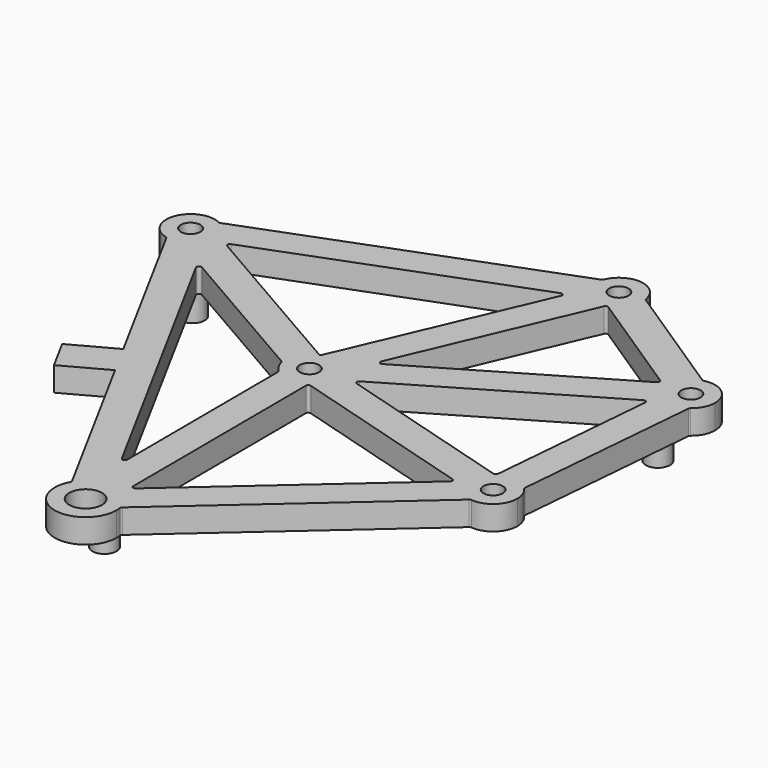
from build123d import *

# Parameters (mm, degrees)
F1_R        = 0.8
F1_R_2      = 1.35
F2_DEPTH    = 2
F3_R        = 1
F4_DEPTH    = 5
F5_T1_DEPTH = 2


# Not quite as in the source:
# - a fillet or chamfer that OpenCascade refuses, or shapes differently, is made with other operations: its cross-section is extruded or revolved along the edge and cut away or added


with BuildPart() as f2:
    # F1 (on Top) → F2 (new body)
    with BuildSketch(Plane.XY):
        with BuildLine():
            ThreePointArc((5.1588517672, 41.7551647468), (5.8189357702, 41.1743283067), (6.1661273036, 40.3665288884))
            Line((6.1661273036, 40.3665288884), (7.2214972283, 39.7576616241))
            Line((7.2214972283, 39.7576616241), (28.9007343827, 47.9973716865))
            Line((28.9007343827, 47.9973716865), (29.5069198348, 49.4140747655))
            ThreePointArc((29.5069198348, 49.4140747655), (29.3032782438, 50.1855350347), (29.4174253255, 50.9752129996))
            Line((29.4174253255, 50.9752129996), (5.1588517672, 41.7551647468))
        make_face()
        with BuildLine():
            Line((43.2422348913, 44.0206504324), (33.2838919458, 50.5533234047))
            ThreePointArc((33.2838919458, 50.5533234047), (33.2959689241, 50.4269175094), (33.3, 50.3))
            ThreePointArc((33.3, 50.3), (32.9116112847, 49.1156398068), (31.8972909329, 48.3912717476))
            Line((31.8972909329, 48.3912717476), (31.8846447163, 48.361716545))
            Line((31.8846447163, 48.361716545), (41.3390492003, 42.1596272035))
            Line((41.3390492003, 42.1596272035), (41.8307045309, 42.4491065103))
            ThreePointArc((41.8307045309, 42.4491065103), (42.3120664109, 43.4364331761), (43.2422348913, 44.0206504324))
        make_face()
        with BuildLine():
            Line((43.6267783824, 25.1015361028), (44.9634471469, 40.4732268946))
            ThreePointArc((44.9634471469, 40.4732268946), (44.0887539119, 40.1209544779), (43.1498718292, 40.2086160195))
            Line((43.1498718292, 40.2086160195), (42.2864184602, 39.7002275873))
            Line((42.2864184602, 39.7002275873), (41.0423751405, 25.3937294107))
            Line((41.0423751405, 25.3937294107), (41.1068738191, 25.3748358584))
            ThreePointArc((41.1068738191, 25.3748358584), (42.4156481787, 25.6883399767), (43.6267783824, 25.1015361028))
        make_face()
        with BuildLine():
            Line((23.7876337156, 9.1717796898), (23.790532231, 8.4993241145))
            ThreePointArc((23.790532231, 8.4993241145), (24.5837459945, 7.769864834), (25.0048179717, 6.7778984503))
            Line((25.0048179717, 6.7778984503), (41.9214502868, 21.7194924748))
            ThreePointArc((41.9214502868, 21.7194924748), (40.9992832251, 22.1005378321), (40.3759708626, 22.8796843864))
            Line((40.3759708626, 22.8796843864), (39.5736067493, 23.1147203388))
            Line((39.5736067493, 23.1147203388), (23.7876337156, 9.1717796898))
        make_face()
        with BuildLine():
            ThreePointArc((6.0825746745, 39.3247870004), (6.1704249985, 39.6573262113), (6.2, 40))
            ThreePointArc((6.2, 40), (6.1915138221, 40.184045365), (6.1661273036, 40.3665288884))
            ThreePointArc((6.1661273036, 40.3665288884), (5.8189357702, 41.1743283067), (5.1588517672, 41.7551647468))
            ThreePointArc((5.1588517672, 41.7551647468), (2.3247456616, 40.6952849534), (3.782863546, 38.0439843613))
            ThreePointArc((3.782863546, 38.0439843613), (4.3297316575, 38.004212011), (4.8668489245, 38.1144463646))
            ThreePointArc((4.8668489245, 38.1144463646), (5.5958497172, 38.5676580133), (6.0677200026, 39.2847224372))
            ThreePointArc((6.0677200026, 39.2847224372), (6.0752543384, 39.3047150466), (6.0825746745, 39.3247870004))
        make_face()
        with Locations((4.2, 40)):
            Circle(F1_R, mode=Mode.SUBTRACT)
        with BuildLine():
            ThreePointArc((33.2838919458, 50.5533234047), (31.5169424001, 52.2881991839), (29.4174253255, 50.9752129996))
            ThreePointArc((29.4174253255, 50.9752129996), (29.3032782438, 50.1855350347), (29.5069198348, 49.4140747655))
            ThreePointArc((29.5069198348, 49.4140747655), (29.8570250617, 48.9151450158), (30.3411482328, 48.5448352532))
            ThreePointArc((30.3411482328, 48.5448352532), (31.0830575999, 48.3118008161), (31.8577651087, 48.3793495676))
            ThreePointArc((31.8577651087, 48.3793495676), (31.8775587843, 48.3852086666), (31.8972909329, 48.3912717476))
            ThreePointArc((31.8972909329, 48.3912717476), (32.9116112847, 49.1156398068), (33.3, 50.3))
            ThreePointArc((33.3, 50.3), (33.2959689241, 50.4269175094), (33.2838919458, 50.5533234047))
        make_face()
        with Locations((31.3, 50.3)):
            Circle(F1_R, mode=Mode.SUBTRACT)
        with BuildLine():
            ThreePointArc((45.8, 42.1), (45.0009308437, 43.699301444), (43.2422348913, 44.0206504324))
            ThreePointArc((43.2422348913, 44.0206504324), (42.3120664109, 43.4364331761), (41.8307045309, 42.4491065103))
            ThreePointArc((41.8307045309, 42.4491065103), (41.8005868024, 42.1484444539), (41.8161080542, 41.8466765953))
            ThreePointArc((41.8161080542, 41.8466765953), (42.0006206287, 41.2269399345), (42.3732216176, 40.6984638972))
            ThreePointArc((42.3732216176, 40.6984638972), (42.7330543859, 40.4083655665), (43.1498718292, 40.2086160195))
            ThreePointArc((43.1498718292, 40.2086160195), (44.0887539119, 40.1209544779), (44.9634471469, 40.4732268946))
            ThreePointArc((44.9634471469, 40.4732268946), (45.578608205, 41.1853673671), (45.8, 42.1))
        make_face()
        with Locations((43.8, 42.1)):
            Circle(F1_R, mode=Mode.SUBTRACT)
        with BuildLine():
            ThreePointArc((44.2, 23.7), (44.0511559584, 24.4571140057), (43.6267783824, 25.1015361028))
            ThreePointArc((43.6267783824, 25.1015361028), (42.4156481787, 25.6883399767), (41.1068738191, 25.3748358584))
            ThreePointArc((41.1068738191, 25.3748358584), (41.071457443, 25.351178881), (41.0365528531, 25.3267731054))
            ThreePointArc((41.0365528531, 25.3267731054), (40.4141774879, 24.6004654104), (40.2002527524, 23.6682046258))
            ThreePointArc((40.2002527524, 23.6682046258), (40.2478838399, 23.2649798885), (40.3759708626, 22.8796843864))
            ThreePointArc((40.3759708626, 22.8796843864), (40.9992832251, 22.1005378321), (41.9214502868, 21.7194924748))
            ThreePointArc((41.9214502868, 21.7194924748), (43.512040505, 22.1905134273), (44.2, 23.7))
        make_face()
        with Locations((42.2, 23.7)):
            Circle(F1_R, mode=Mode.SUBTRACT)
        with BuildLine():
            ThreePointArc((22.5955597255, 8.8482088491), (21.8669162755, 8.7701629496), (21.1905563835, 8.4881173221))
            ThreePointArc((21.1905563835, 8.4881173221), (20.6960652476, 8.1023094654), (20.3107032689, 7.6074707733))
            ThreePointArc((20.3107032689, 7.6074707733), (21.8218431835, 3.8418292711), (25.05, 6.3))
            ThreePointArc((25.05, 6.3), (25.0386793641, 6.5400147623), (25.0048179717, 6.7778984503))
            ThreePointArc((25.0048179717, 6.7778984503), (24.5837459945, 7.769864834), (23.790532231, 8.4993241145))
            ThreePointArc((23.790532231, 8.4993241145), (23.5432842899, 8.6268128181), (23.2836204373, 8.7266106013))
            ThreePointArc((23.2836204373, 8.7266106013), (22.9437746873, 8.8110882157), (22.5955597255, 8.8482088491))
        make_face()
        with Locations((22.5, 6.3)):
            Circle(F1_R_2, mode=Mode.SUBTRACT)
        with BuildLine():
            Line((7.2214972283, 39.7576616241), (6.0825746745, 39.3247870004))
            ThreePointArc((6.0825746745, 39.3247870004), (6.0752543384, 39.3047150466), (6.0677200026, 39.2847224372))
            Line((6.0677200026, 39.2847224372), (7.5409732288, 36.5716823429))
            Line((7.5409732288, 36.5716823429), (20.4338726964, 29.1334711116))
            ThreePointArc((20.4338726964, 29.1334711116), (20.6676288279, 30.499444907), (21.7331510755, 31.3855536354))
            Line((21.7331510755, 31.3855536354), (7.2214972283, 39.7576616241))
        make_face()
        with BuildLine():
            ThreePointArc((6.1661273036, 40.3665288884), (6.1915138221, 40.184045365), (6.2, 40))
            ThreePointArc((6.2, 40), (6.1704249985, 39.6573262113), (6.0825746745, 39.3247870004))
            Line((6.0825746745, 39.3247870004), (7.2214972283, 39.7576616241))
            Line((7.2214972283, 39.7576616241), (6.1661273036, 40.3665288884))
        make_face()
        with BuildLine():
            Line((7.5409732288, 36.5716823429), (6.0677200026, 39.2847224372))
            ThreePointArc((6.0677200026, 39.2847224372), (5.5958497172, 38.5676580133), (4.8668489245, 38.1144463646))
            Line((4.8668489245, 38.1144463646), (7.5409732288, 36.5716823429))
        make_face()
        with BuildLine():
            ThreePointArc((4.8668489245, 38.1144463646), (4.3297316575, 38.004212011), (3.782863546, 38.0439843613))
            Line((3.782863546, 38.0439843613), (11.3309729791, 24.1439139846))
            Line((11.3309729791, 24.1439139846), (12.7625938358, 21.5075411501))
            Line((12.7625938358, 21.5075411501), (20.3107032689, 7.6074707733))
            ThreePointArc((20.3107032689, 7.6074707733), (20.6960652476, 8.1023094654), (21.1905563835, 8.4881173221))
            Line((21.1905563835, 8.4881173221), (21.1777502182, 11.4591476685))
            Line((21.1777502182, 11.4591476685), (7.5409732288, 36.5716823429))
            Line((7.5409732288, 36.5716823429), (4.8668489245, 38.1144463646))
        make_face()
        with BuildLine():
            Line((22.5955597255, 8.8482088491), (21.1777502182, 11.4591476685))
            Line((21.1777502182, 11.4591476685), (21.1905563835, 8.4881173221))
            ThreePointArc((21.1905563835, 8.4881173221), (21.8669162755, 8.7701629496), (22.5955597255, 8.8482088491))
        make_face()
        with BuildLine():
            Line((23.7876337156, 9.1717796898), (23.2836204373, 8.7266106013))
            ThreePointArc((23.2836204373, 8.7266106013), (23.5432842899, 8.6268128181), (23.790532231, 8.4993241145))
            Line((23.790532231, 8.4993241145), (23.7876337156, 9.1717796898))
        make_face()
        with BuildLine():
            Line((21.1065631723, 27.9745423071), (21.1777502182, 11.4591476685))
            Line((21.1777502182, 11.4591476685), (22.5955597255, 8.8482088491))
            ThreePointArc((22.5955597255, 8.8482088491), (22.9437746873, 8.8110882157), (23.2836204373, 8.7266106013))
            Line((23.2836204373, 8.7266106013), (23.7876337156, 9.1717796898))
            Line((23.7876337156, 9.1717796898), (23.7075018728, 27.7623672218))
            Line((23.7075018728, 27.7623672218), (23.4931261809, 27.8251641416))
            ThreePointArc((23.4931261809, 27.8251641416), (22.2750618238, 27.5039062016), (21.1065631723, 27.9745423071))
        make_face()
        with BuildLine():
            Line((40.2002527524, 23.6682046258), (39.5736067493, 23.1147203388))
            Line((39.5736067493, 23.1147203388), (40.3759708626, 22.8796843864))
            ThreePointArc((40.3759708626, 22.8796843864), (40.2478838399, 23.2649798885), (40.2002527524, 23.6682046258))
        make_face()
        with BuildLine():
            ThreePointArc((41.0365528531, 25.3267731054), (41.071457443, 25.351178881), (41.1068738191, 25.3748358584))
            Line((41.1068738191, 25.3748358584), (41.0423751405, 25.3937294107))
            Line((41.0423751405, 25.3937294107), (41.0365528531, 25.3267731054))
        make_face()
        with BuildLine():
            Line((29.5069198348, 49.4140747655), (28.9007343827, 47.9973716865))
            Line((28.9007343827, 47.9973716865), (30.3411482328, 48.5448352532))
            ThreePointArc((30.3411482328, 48.5448352532), (29.8570250617, 48.9151450158), (29.5069198348, 49.4140747655))
        make_face()
        with BuildLine():
            ThreePointArc((31.8972909329, 48.3912717476), (31.8775587843, 48.3852086666), (31.8577651087, 48.3793495676))
            Line((31.8577651087, 48.3793495676), (31.8846447163, 48.361716545))
            Line((31.8846447163, 48.361716545), (31.8972909329, 48.3912717476))
        make_face()
        with BuildLine():
            ThreePointArc((23.7065390199, 27.9857490995), (23.602516175, 27.9018902263), (23.4931261809, 27.8251641416))
            Line((23.4931261809, 27.8251641416), (23.7075018728, 27.7623672218))
            Line((23.7075018728, 27.7623672218), (23.7065390199, 27.9857490995))
        make_face()
        with BuildLine():
            Line((30.3411482328, 48.5448352532), (28.9007343827, 47.9973716865))
            Line((28.9007343827, 47.9973716865), (21.8027090671, 31.4087282524))
            ThreePointArc((21.8027090671, 31.4087282524), (22.4278055637, 31.4998067033), (23.0501281708, 31.3913839805))
            Line((23.0501281708, 31.3913839805), (25.1531087237, 32.6295874836))
            Line((25.1531087237, 32.6295874836), (31.8846447163, 48.361716545))
            Line((31.8846447163, 48.361716545), (31.8577651087, 48.3793495676))
            ThreePointArc((31.8577651087, 48.3793495676), (31.0830575999, 48.3118008161), (30.3411482328, 48.5448352532))
        make_face()
        with BuildLine():
            Line((25.1531087237, 32.6295874836), (23.0501281708, 31.3913839805))
            ThreePointArc((23.0501281708, 31.3913839805), (23.7210047561, 31.0016479062), (24.1930801652, 30.3859252345))
            Line((24.1930801652, 30.3859252345), (25.1531087237, 32.6295874836))
        make_face()
        with BuildLine():
            ThreePointArc((21.8027090671, 31.4087282524), (21.7678238691, 31.397459707), (21.7331510755, 31.3855536354))
            ThreePointArc((21.7331510755, 31.3855536354), (20.6676288279, 30.499444907), (20.4338726964, 29.1334711116))
            ThreePointArc((20.4338726964, 29.1334711116), (20.6702692189, 28.4959923182), (21.1065631723, 27.9745423071))
            ThreePointArc((21.1065631723, 27.9745423071), (22.2750618238, 27.5039062016), (23.4931261809, 27.8251641416))
            ThreePointArc((23.4931261809, 27.8251641416), (23.602516175, 27.9018902263), (23.7065390199, 27.9857490995))
            ThreePointArc((23.7065390199, 27.9857490995), (24.138437017, 28.5111437224), (24.3692954691, 29.1508934897))
            ThreePointArc((24.3692954691, 29.1508934897), (24.3923090797, 29.3247729161), (24.4, 29.5))
            ThreePointArc((24.4, 29.5), (24.3555124999, 29.9194888111), (24.2240291374, 30.3203156136))
            ThreePointArc((24.2240291374, 30.3203156136), (24.208852145, 30.353260756), (24.1930801652, 30.3859252345))
            ThreePointArc((24.1930801652, 30.3859252345), (23.7210047561, 31.0016479062), (23.0501281708, 31.3913839805))
            ThreePointArc((23.0501281708, 31.3913839805), (22.4278055637, 31.4998067033), (21.8027090671, 31.4087282524))
        make_face()
        with Locations((22.4, 29.5)):
            Circle(F1_R, mode=Mode.SUBTRACT)
        with BuildLine():
            ThreePointArc((24.3692954691, 29.1508934897), (24.138437017, 28.5111437224), (23.7065390199, 27.9857490995))
            Line((23.7065390199, 27.9857490995), (23.7075018728, 27.7623672218))
            Line((23.7075018728, 27.7623672218), (39.5736067493, 23.1147203388))
            Line((39.5736067493, 23.1147203388), (40.2002527524, 23.6682046258))
            ThreePointArc((40.2002527524, 23.6682046258), (40.4141774879, 24.6004654104), (41.0365528531, 25.3267731054))
            Line((41.0365528531, 25.3267731054), (41.0423751405, 25.3937294107))
            Line((41.0423751405, 25.3937294107), (25.6473390591, 29.9033864446))
            Line((25.6473390591, 29.9033864446), (24.3692954691, 29.1508934897))
        make_face()
        with BuildLine():
            Line((25.6473390591, 29.9033864446), (24.2240291374, 30.3203156136))
            ThreePointArc((24.2240291374, 30.3203156136), (24.3555124999, 29.9194888111), (24.4, 29.5))
            ThreePointArc((24.4, 29.5), (24.3923090797, 29.3247729161), (24.3692954691, 29.1508934897))
            Line((24.3692954691, 29.1508934897), (25.6473390591, 29.9033864446))
        make_face()
        with BuildLine():
            Line((25.1531087237, 32.6295874836), (24.1930801652, 30.3859252345))
            ThreePointArc((24.1930801652, 30.3859252345), (24.208852145, 30.353260756), (24.2240291374, 30.3203156136))
            Line((24.2240291374, 30.3203156136), (25.6473390591, 29.9033864446))
            Line((25.6473390591, 29.9033864446), (42.2864184602, 39.7002275873))
            Line((42.2864184602, 39.7002275873), (42.3732216176, 40.6984638972))
            ThreePointArc((42.3732216176, 40.6984638972), (42.0006206287, 41.2269399345), (41.8161080542, 41.8466765953))
            Line((41.8161080542, 41.8466765953), (41.3390492003, 42.1596272035))
            Line((41.3390492003, 42.1596272035), (25.1531087237, 32.6295874836))
        make_face()
        with BuildLine():
            ThreePointArc((41.8161080542, 41.8466765953), (41.8005868024, 42.1484444539), (41.8307045309, 42.4491065103))
            Line((41.8307045309, 42.4491065103), (41.3390492003, 42.1596272035))
            Line((41.3390492003, 42.1596272035), (41.8161080542, 41.8466765953))
        make_face()
        with BuildLine():
            Line((42.2864184602, 39.7002275873), (43.1498718292, 40.2086160195))
            ThreePointArc((43.1498718292, 40.2086160195), (42.7330543859, 40.4083655665), (42.3732216176, 40.6984638972))
            Line((42.3732216176, 40.6984638972), (42.2864184602, 39.7002275873))
        make_face()
        Polygon((12.7625938358, 21.5075411501), (11.3309729791, 24.1439139846), (7.8158091997, 22.2350861756), (9.2474300564, 19.5987133411), align=None)
    extrude(amount=-F2_DEPTH)

    # F3 (on face) → F4 (join)
    with BuildSketch(Plane.XY):
        with Locations((21.6236830238, 9.3353357393)):
            Circle(F3_R)
        with Locations((5.9410208844, 38.0202536185)):
            Circle(F3_R)
        with Locations((41.960581314, 40.9868787588)):
            Circle(F3_R)
    extrude(amount=-F4_DEPTH)

    # F5: fillet of radius 0.2 on 26 edges, made by hand

    # F5_s2 → F5_t1 (join)
    with BuildSketch(Plane.XY.offset(-2)):
        with BuildLine():
            ThreePointArc((7.6152873474, 39.9073309314), (7.4869831486, 39.736368397), (7.586398465, 39.5471416799))
            Line((7.586398465, 39.5471416799), (7.2214972283, 39.7576616241))
            Line((7.2214972283, 39.7576616241), (7.6152873474, 39.9073309314))
        make_face()
        with BuildLine():
            ThreePointArc((8.1549136009, 36.2174859744), (7.9153841385, 36.1874830559), (7.8792109212, 35.9488074668))
            Line((7.8792109212, 35.9488074668), (7.5409732288, 36.5716823429))
            Line((7.5409732288, 36.5716823429), (8.1549136009, 36.2174859744))
        make_face()
        with BuildLine():
            ThreePointArc((20.7985689859, 12.157421304), (21.0239808003, 12.0591244239), (21.174325317, 12.2537247554))
            Line((21.174325317, 12.2537247554), (21.1777502182, 11.4591476685))
            Line((21.1777502182, 11.4591476685), (20.7985689859, 12.157421304))
        make_face()
        with BuildLine():
            ThreePointArc((23.7857330682, 9.6127298888), (23.9039049915, 9.4310968268), (24.1181310207, 9.463691015))
            Line((24.1181310207, 9.463691015), (23.7876337156, 9.1717796898))
            Line((23.7876337156, 9.1717796898), (23.7857330682, 9.6127298888))
        make_face()
        with BuildLine():
            ThreePointArc((20.2576640938, 7.7051440082), (20.2819058756, 7.6098108546), (20.2577672936, 7.5144515183))
            ThreePointArc((20.2577672936, 7.5144515183), (20.2837472088, 7.5612389011), (20.3107032689, 7.6074707733))
            Line((20.3107032689, 7.6074707733), (20.2576640938, 7.7051440082))
        make_face()
        with BuildLine():
            ThreePointArc((25.0881216817, 6.8514763464), (25.0326730948, 6.7702265564), (25.0226653835, 6.6723699273))
            ThreePointArc((25.0226653835, 6.6723699273), (25.0142953862, 6.7252278342), (25.0048179717, 6.7778984503))
            Line((25.0048179717, 6.7778984503), (25.0881216817, 6.8514763464))
        make_face()
        with BuildLine():
            ThreePointArc((21.0426824665, 28.0310925443), (21.090007357, 27.9647639806), (21.1069488553, 27.8850638597))
            Line((21.1069488553, 27.8850638597), (21.1065631723, 27.9745423071))
            ThreePointArc((21.1065631723, 27.9745423071), (21.0743212482, 28.0024767625), (21.0426824665, 28.0310925443))
        make_face()
        with BuildLine():
            ThreePointArc((20.356367035, 29.1781859163), (20.4171704433, 29.1239450721), (20.4512932221, 29.0499534537))
            ThreePointArc((20.4512932221, 29.0499534537), (20.442137576, 29.0916193824), (20.4338726964, 29.1334711116))
            Line((20.4338726964, 29.1334711116), (20.356367035, 29.1781859163))
        make_face()
        with BuildLine():
            ThreePointArc((3.6998231735, 38.0635539919), (3.77290973, 38.0275334575), (3.8255636798, 37.9653507815))
            Line((3.8255636798, 37.9653507815), (3.782863546, 38.0439843613))
            ThreePointArc((3.782863546, 38.0439843613), (3.7412389988, 38.0533263387), (3.6998231735, 38.0635539919))
        make_face()
        with BuildLine():
            ThreePointArc((5.2424934778, 41.7869547697), (5.1620285352, 41.7741283656), (5.0831253359, 41.7944608218))
            ThreePointArc((5.0831253359, 41.7944608218), (5.1211981098, 41.7752166185), (5.1588517672, 41.7551647468))
            Line((5.1588517672, 41.7551647468), (5.2424934778, 41.7869547697))
        make_face()
        with BuildLine():
            ThreePointArc((29.3337836149, 50.9434229768), (29.4024548833, 50.9872793392), (29.4479345515, 51.0548864647))
            ThreePointArc((29.4479345515, 51.0548864647), (29.4322550556, 51.0152124318), (29.4174253255, 50.9752129996))
            Line((29.4174253255, 50.9752129996), (29.3337836149, 50.9434229768))
        make_face()
        with BuildLine():
            ThreePointArc((28.4605609872, 47.8300733111), (28.6759140893, 47.7816066752), (28.7154912953, 47.5644440215))
            Line((28.7154912953, 47.5644440215), (28.9007343827, 47.9973716865))
            Line((28.9007343827, 47.9973716865), (28.4605609872, 47.8300733111))
        make_face()
        with BuildLine():
            ThreePointArc((31.7907153575, 48.1421962456), (31.9168341789, 48.2549982237), (32.0842921217, 48.230747847))
            Line((32.0842921217, 48.230747847), (31.8846447163, 48.361716545))
            Line((31.8846447163, 48.361716545), (31.7907153575, 48.1421962456))
        make_face()
        with BuildLine():
            ThreePointArc((33.2712832298, 50.637701685), (33.3011123586, 50.5618772384), (33.3587094883, 50.5042430968))
            Line((33.3587094883, 50.5042430968), (33.2838919458, 50.5533234047))
            ThreePointArc((33.2838919458, 50.5533234047), (33.2780375605, 50.5955797846), (33.2712832298, 50.637701685))
        make_face()
        with BuildLine():
            ThreePointArc((43.1674173488, 44.0697307403), (43.2432226177, 44.0398529085), (43.324654012, 44.0426904518))
            ThreePointArc((43.324654012, 44.0426904518), (43.2833269166, 44.0321099671), (43.2422348913, 44.0206504324))
            Line((43.2422348913, 44.0206504324), (43.1674173488, 44.0697307403))
        make_face()
        with BuildLine():
            ThreePointArc((45.0317670082, 40.5243255293), (44.9791416551, 40.4621186499), (44.9556955913, 40.3840840055))
            Line((44.9556955913, 40.3840840055), (44.9634471469, 40.4732268946))
            ThreePointArc((44.9634471469, 40.4732268946), (44.9978795765, 40.4984118756), (45.0317670082, 40.5243255293))
        make_face()
        with BuildLine():
            ThreePointArc((42.2528078794, 39.3137059082), (42.1602543232, 39.5001952749), (41.9520853542, 39.5033772539))
            Line((41.9520853542, 39.5033772539), (42.2864184602, 39.7002275873))
            Line((42.2864184602, 39.7002275873), (42.2528078794, 39.3137059082))
        make_face()
        with BuildLine():
            ThreePointArc((41.0619157925, 41.996455197), (41.1603827047, 42.163956174), (41.0701434494, 42.3360293761))
            Line((41.0701434494, 42.3360293761), (41.3390492003, 42.1596272035))
            Line((41.3390492003, 42.1596272035), (41.0619157925, 41.996455197))
        make_face()
        with BuildLine():
            ThreePointArc((43.634529938, 25.190678992), (43.6441546963, 25.1097686239), (43.6852527778, 25.0394118806))
            ThreePointArc((43.6852527778, 25.0394118806), (43.6563468764, 25.0707858242), (43.6267783824, 25.1015361028))
            Line((43.6267783824, 25.1015361028), (43.634529938, 25.190678992))
        make_face()
        with BuildLine():
            ThreePointArc((42.0061681452, 21.7094148569), (41.9251626725, 21.7006263973), (41.8543851494, 21.6602572772))
            Line((41.8543851494, 21.6602572772), (41.9214502868, 21.7194924748))
            ThreePointArc((41.9214502868, 21.7194924748), (41.9637554741, 21.7140018822), (42.0061681452, 21.7094148569))
        make_face()
        with BuildLine():
            ThreePointArc((39.3019460595, 22.8747763793), (39.3647578651, 23.0681793251), (39.2257695535, 23.2166120426))
            Line((39.2257695535, 23.2166120426), (39.5736067493, 23.1147203388))
            Line((39.5736067493, 23.1147203388), (39.3019460595, 22.8747763793))
        make_face()
        with BuildLine():
            ThreePointArc((40.8080557039, 25.4623684376), (40.977133264, 25.4891852781), (41.0635271259, 25.6369772429))
            Line((41.0635271259, 25.6369772429), (41.0423751405, 25.3937294107))
            Line((41.0423751405, 25.3937294107), (40.8080557039, 25.4623684376))
        make_face()
        with BuildLine():
            ThreePointArc((21.8379089426, 31.4909931299), (21.7912680279, 31.4241818381), (21.7218493116, 31.381518441))
            ThreePointArc((21.7218493116, 31.381518441), (21.7621340848, 31.3955545559), (21.8027090671, 31.4087282524))
            Line((21.8027090671, 31.4087282524), (21.8379089426, 31.4909931299))
        make_face()
        with BuildLine():
            ThreePointArc((25.3927892122, 33.1897396363), (25.4445634364, 32.9608976905), (25.6781383196, 32.9387170587))
            Line((25.6781383196, 32.9387170587), (25.1531087237, 32.6295874836))
            Line((25.1531087237, 32.6295874836), (25.3927892122, 33.1897396363))
        make_face()
        with BuildLine():
            ThreePointArc((26.0907063793, 29.773511169), (25.9484551281, 29.9407912669), (26.0454552761, 30.13779132))
            Line((26.0454552761, 30.13779132), (25.6473390591, 29.9033864446))
            Line((25.6473390591, 29.9033864446), (26.0907063793, 29.773511169))
        make_face()
        with BuildLine():
            ThreePointArc((23.708657865, 27.4941770411), (23.7884043896, 27.6548500794), (23.9648793114, 27.6869738307))
            Line((23.9648793114, 27.6869738307), (23.7075018728, 27.7623672218))
            Line((23.7075018728, 27.7623672218), (23.708657865, 27.4941770411))
        make_face()
    extrude(amount=F5_T1_DEPTH)


solid = f2.part
